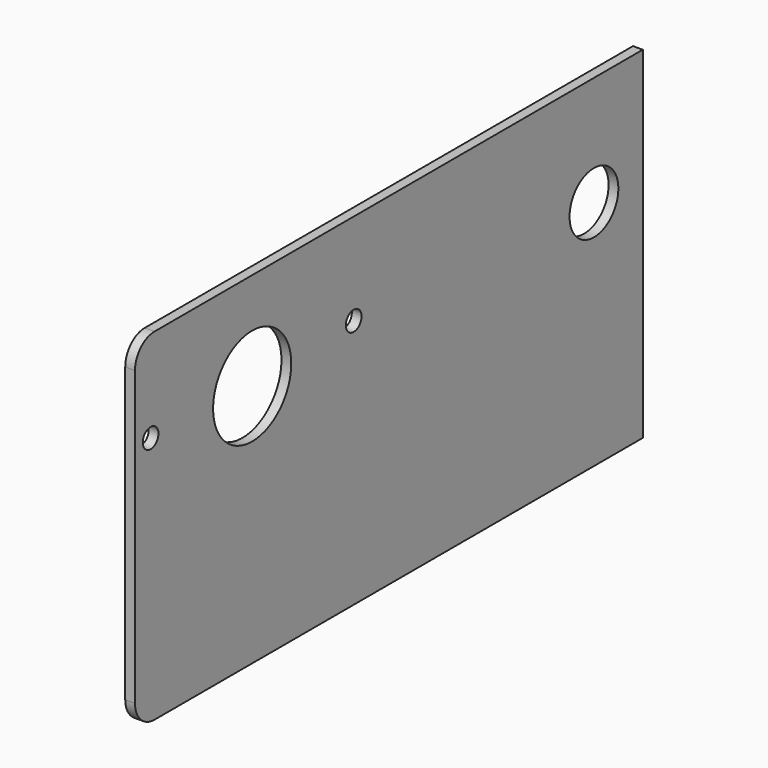
from build123d import *

# Parameters (mm, degrees)
F1_DEPTH = 2.54
F2_R     = 12.7
F3_DEPTH = 2.541
F2_R_2   = 7.9375
F4_DEPTH = 25.4
F5_R     = 2.5527
F6_DEPTH = 25.4


# Not quite as in the source:
# - a feature names something its author has since deleted; it is built from what else it names


with BuildPart() as f1:
    # F0 (on Right) → F1 (new body)
    with BuildSketch(Plane.YZ):
        with BuildLine():
            ThreePointArc((0, 6.35), (1.8598719395, 1.8598719395), (6.35, 0))
            Line((6.35, 0), (165.1, 0))
            Line((165.1, 0), (165.1, 88.9))
            Line((165.1, 88.9), (6.35, 88.9))
            ThreePointArc((6.35, 88.9), (1.8598719395, 87.0401280605), (0, 82.55))
            Line((0, 82.55), (0, 6.35))
        make_face()
    extrude(amount=F1_DEPTH)

    # F2 (on face) → F3 (cut, through all)
    with BuildSketch(Plane.YZ.offset(2.54)):
        with Locations((38.1, 63.5)):
            Circle(F2_R)
    extrude(amount=-F3_DEPTH, mode=Mode.SUBTRACT)

    # F2 (on face) → F4 (cut)
    with BuildSketch(Plane.YZ.offset(2.54)):
        with Locations((38.1, 63.5)):
            Circle(F2_R)
        with Locations((149.225, 60.325)):
            Circle(F2_R_2)
    extrude(amount=-F4_DEPTH, mode=Mode.SUBTRACT)

    # F5 (on face) → F6 (cut)
    with BuildSketch(Plane.YZ.offset(2.54)):
        with Locations((5.08, 65.024)):
            Circle(F5_R)
        with Locations((71.12, 65.024)):
            Circle(F5_R)
    extrude(amount=-F6_DEPTH, mode=Mode.SUBTRACT)


solid = f1.part
